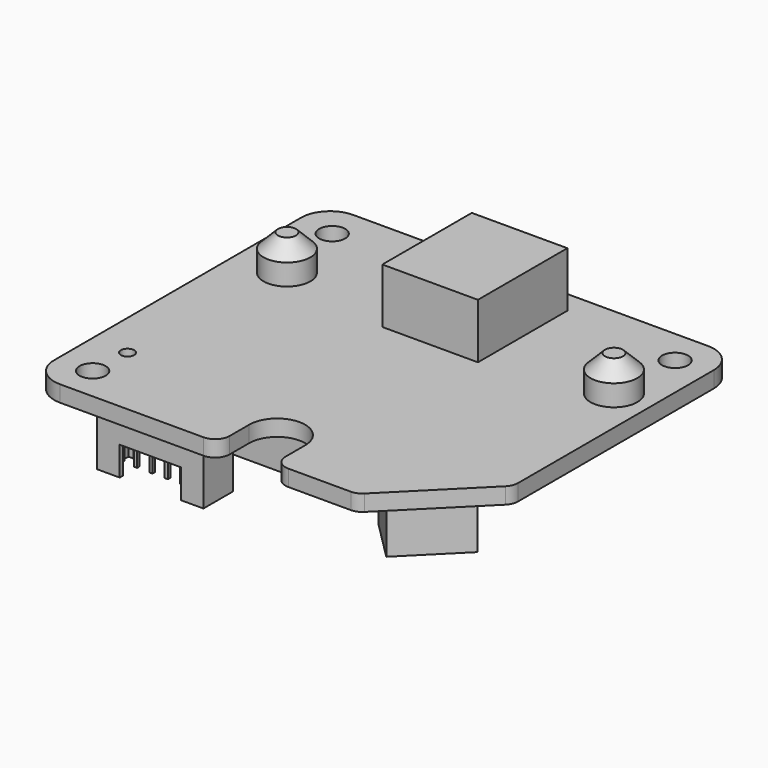
from build123d import *

# Parameters (mm, degrees)
F0_R      = 1.143
F0_R_2    = 0.5842
F1_DEPTH  = 1.4224
F2_W      = 8.382
F2_H      = 9.8044
F3_DEPTH  = 4.826
F2_R      = 2.0574
F4_DEPTH  = 3.1242
F5_SIZE   = 1.27
F6_W      = 8.4328
F6_H      = 9.7282
F7_DEPTH  = 4.5974
F8_DEPTH  = 4.5212
F9_W      = 5.3594
F9_H      = 0.381
F10_DEPTH = 2.1844
F11_DEPTH = 4.7244
F9_W_2    = 7.3914
F9_H_2    = 0.4572
F12_DEPTH = 3.2258
F13_W     = 0.2794
F13_H     = 0.2794
F14_DEPTH = 1.905


with BuildPart() as f1:
    # F0 (on Top) → F1 (new body)
    with BuildSketch(Plane.XY):
        with BuildLine():
            Line((15.5575, 16.0782), (-15.5575, 16.0782))
            ThreePointArc((-15.5575, 16.0782), (-17.3535512242, 15.3342512242), (-18.0975, 13.5382))
            Line((-18.0975, 13.5382), (-18.0975, -13.5382))
            ThreePointArc((-18.0975, -13.5382), (-17.3535512242, -15.3342512242), (-15.5575, -16.0782))
            Line((-15.5575, -16.0782), (-2.9591, -16.0782))
            ThreePointArc((-2.9591, -16.0782), (-2.0610743879, -15.7062256121), (-1.6891, -14.8082))
            Line((-1.6891, -14.8082), (-1.6891, -12.6619))
            ThreePointArc((-1.6891, -12.6619), (0.762, -10.2108), (3.2131, -12.6619))
            Line((3.2131, -12.6619), (3.2131, -14.8082))
            ThreePointArc((3.2131, -14.8082), (3.5850743879, -15.7062256121), (4.4831, -16.0782))
            Line((4.4831, -16.0782), (9.9514487758, -16.0782))
            ThreePointArc((9.9514487758, -16.0782), (10.4374567349, -15.9815270063), (10.8494743879, -15.7062256121))
            Line((10.8494743879, -15.7062256121), (17.7255256121, -8.8301743879))
            ThreePointArc((17.7255256121, -8.8301743879), (18.0008270063, -8.4181567349), (18.0975, -7.9321487758))
            Line((18.0975, -7.9321487758), (18.0975, 13.5382))
            ThreePointArc((18.0975, 13.5382), (17.3535512242, 15.3342512242), (15.5575, 16.0782))
        make_face()
        with Locations((-15.0495, -13.1318)):
            Circle(F0_R, mode=Mode.SUBTRACT)
        with Locations((-14.8717, -9.525)):
            Circle(F0_R_2, mode=Mode.SUBTRACT)
        with Locations((-14.9479, 13.0048)):
            Circle(F0_R, mode=Mode.SUBTRACT)
        with Locations((15.1257, 13.0048)):
            Circle(F0_R, mode=Mode.SUBTRACT)
    extrude(amount=F1_DEPTH)

    # F2 (on face) → F4 (join)
    with BuildSketch(Plane.XY.offset(1.4224)):
        with Locations((-13.7541, 6.5532)):
            Circle(F2_R)
        with Locations((14.9225, 6.5532)):
            Circle(F2_R)
    extrude(amount=F4_DEPTH)

    # F5
    f5_edges = [f1.edges().sort_by_distance(p)[0] for p in [
        (-15.8115, 6.5532, 4.5466),
        (12.8651, 6.5532, 4.5466),
    ]]
    chamfer(f5_edges, length=F5_SIZE)


with BuildPart() as f3:
    # F2 (on face) → F3 (new body)
    with BuildSketch(Plane.XY.offset(1.4224)):
        with Locations((0.5715, 9.2456)):
            Rectangle(F2_W, F2_H)
    extrude(amount=F3_DEPTH)


with BuildPart() as f7:
    # F6 (on face) → F7 (new body)
    with BuildSketch(Plane(origin=(0, 0, 0), x_dir=(1, 0, 0), z_dir=(0, 0, -1))):
        with Locations((1.8161, -7.3533)):
            Rectangle(F6_W, F6_H)
    extrude(amount=F7_DEPTH)


with BuildPart() as f7b:
    # F6 (on face) → F7, piece 2 (new body)
    with BuildSketch(Plane(origin=(0, 0, 0), x_dir=(1, 0, 0), z_dir=(0, 0, -1))):
        with Locations((-4.1783, 2.9083)):
            Rectangle(F6_W, F6_H)
    extrude(amount=F7_DEPTH)


with BuildPart() as f8:
    # F6 (on face) → F8 (new body)
    with BuildSketch(Plane(origin=(0, 0, 0), x_dir=(1, 0, 0), z_dir=(0, 0, -1))):
        Polygon((11.8628308473, 5.3893238113), (15.2034861243, 8.7299790883), (10.7492790883, 13.1841861243), (7.4086238113, 9.8435308473), align=None)
    extrude(amount=F8_DEPTH)


with BuildPart() as f10:
    # F9 (on face) → F10 (new body)
    with BuildSketch(Plane(origin=(0, 0, 0), x_dir=(1, 0, 0), z_dir=(0, 0, -1))):
        Polygon((-12.1031, 12.319), (-4.7117, 12.319), (-4.2545, 12.319), (-4.2545, 12.8778), (-4.0259, 12.8778), (-4.0259, 13.9446), (-4.2545, 13.9446), (-4.2545, 14.732), (-5.7277, 14.732), (-11.0871, 14.732), (-12.5603, 14.732), (-12.5603, 13.9446), (-12.7889, 13.9446), (-12.7889, 12.8778), (-12.5603, 12.8778), (-12.5603, 12.319), align=None)
        with Locations((-8.4074, 14.9225)):
            Rectangle(F9_W, F9_H)
    extrude(amount=F10_DEPTH)

    # F9 (on face) → F11 (join)
    with BuildSketch(Plane(origin=(0, 0, 0), x_dir=(1, 0, 0), z_dir=(0, 0, -1))):
        Polygon((-4.7117, 11.8618), (-3.7465, 11.8618), (-3.7465, 15.113), (-5.7277, 15.113), (-5.7277, 14.732), (-4.2545, 14.732), (-4.2545, 13.9446), (-4.0259, 13.9446), (-4.0259, 12.8778), (-4.2545, 12.8778), (-4.2545, 12.319), (-4.7117, 12.319), align=None)
        Polygon((-13.0683, 11.8618), (-12.1031, 11.8618), (-12.1031, 12.319), (-12.5603, 12.319), (-12.5603, 12.8778), (-12.7889, 12.8778), (-12.7889, 13.9446), (-12.5603, 13.9446), (-12.5603, 14.732), (-11.0871, 14.732), (-11.0871, 15.113), (-13.0683, 15.113), align=None)
    extrude(amount=F11_DEPTH)

    # F9 (on face) → F12 (join)
    with BuildSketch(Plane(origin=(0, 0, 0), x_dir=(1, 0, 0), z_dir=(0, 0, -1))):
        with Locations((-8.4074, 12.0904)):
            Rectangle(F9_W_2, F9_H_2)
    extrude(amount=F12_DEPTH)

    # F13 (on face) → F14 (join)
    with BuildSketch(Plane(origin=(0, 0, -2.1844), x_dir=(1, 0, 0), z_dir=(0, 0, -1))):
        with Locations((-11.7729, 14.0589)):
            Rectangle(F13_W, F13_H)
        with Locations((-10.4267, 14.0589)):
            Rectangle(F13_W, F13_H)
        with Locations((-9.0805, 14.0589)):
            Rectangle(F13_W, F13_H)
        with Locations((-5.0419, 14.0589)):
            Rectangle(F13_W, F13_H)
        with Locations((-6.3881, 14.0589)):
            Rectangle(F13_W, F13_H)
        with Locations((-7.7343, 14.0589)):
            Rectangle(F13_W, F13_H)
    extrude(amount=F14_DEPTH)


solid = Compound([f1.part, f3.part, f7.part, f7b.part, f8.part, f10.part])
